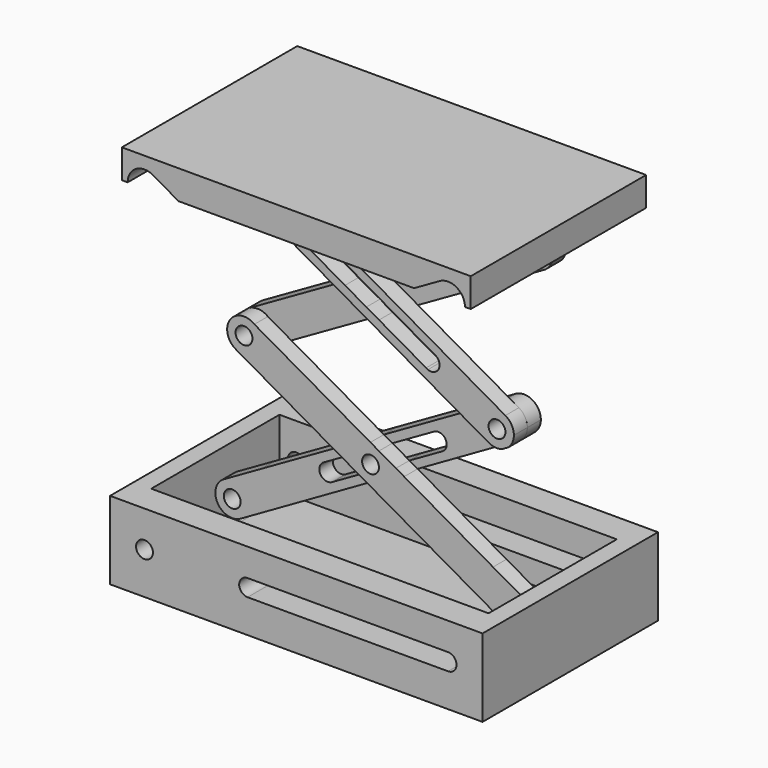
from build123d import *

# Parameters (mm, degrees)
F0_R     = 5
F1_DEPTH = 65
F2_DEPTH = 65
F3_DEPTH = 10
F4_DEPTH = 10
F6_DEPTH = 47.5


# Not quite as in the source:
# - a feature names something its author has since deleted; it is built from what else it names


with BuildPart() as f1:
    # F0 (on Front) → F1 (new body, symmetric)
    with BuildSketch(Plane.XZ):
        with BuildLine():
            Line((-101.2363367384, 45.0652157913), (-79.5725504618, 57.4387013912))
            Line((-79.5725504618, 57.4387013912), (-117.3849242899, 57.4387013912))
            Line((-117.3849242899, 57.4387013912), (-117.3849242899, 11.2442991069))
            Line((-117.3849242899, 11.2442991069), (-6.9597655522, 11.2442991069))
            Line((-6.9597655522, 11.2442991069), (103.4653931856, 11.2442991069))
            Line((103.4653931856, 11.2442991069), (103.4653931856, 57.4387013912))
            Line((103.4653931856, 57.4387013912), (65.6763988632, 57.4387013912))
            Line((65.6763988632, 57.4387013912), (87.9937572054, 44.7127273849))
            ThreePointArc((87.9937572054, 44.7127273849), (91.6870612524, 41.0489903412), (93.0402344479, 36.0258054737))
            ThreePointArc((93.0402344479, 36.0258054737), (87.7852934476, 27.2232822509), (77.54335143, 27.6721070659))
            Line((77.54335143, 27.6721070659), (71.668050416, 31.0258054737))
            Line((71.668050416, 31.0258054737), (-35.829693079, 31.0258054737))
            ThreePointArc((-35.829693079, 31.0258054737), (-40.829693079, 36.0258054737), (-35.829693079, 41.0258054737))
            Line((-35.829693079, 41.0258054737), (54.1491793085, 41.0258054737))
            Line((54.1491793085, 41.0258054737), (25.3956385004, 57.4387013912))
            Line((25.3956385004, 57.4387013912), (-39.4630207883, 57.4387013912))
            Line((-39.4630207883, 57.4387013912), (-91.9890244833, 27.3487245576))
            ThreePointArc((-91.9890244833, 27.3487245576), (-105.4423640429, 30.730003094), (-102.5730303875, 44.3017500052))
            ThreePointArc((-102.5730303875, 44.3017500052), (-101.9193959956, 44.7092417673), (-101.2363367384, 45.0652157913))
        make_face()
        with BuildLine():
            ThreePointArc((93.0402344479, 36.0258054737), (91.6870612524, 41.0489903412), (87.9937572054, 44.7127273849))
            ThreePointArc((87.9937572054, 44.7127273849), (80.4261739109, 45.6780947104), (74.37998041, 41.0258054737))
            Line((74.37998041, 41.0258054737), (83.0402344479, 41.0258054737))
            ThreePointArc((83.0402344479, 41.0258054737), (86.5757683538, 39.5613393797), (88.0402344479, 36.0258054737))
            ThreePointArc((88.0402344479, 36.0258054737), (86.5757683538, 32.4902715678), (83.0402344479, 31.0258054737))
            Line((83.0402344479, 31.0258054737), (74.37998041, 31.0258054737))
            ThreePointArc((74.37998041, 31.0258054737), (75.7657615696, 29.1641697836), (77.54335143, 27.6721070659))
            ThreePointArc((77.54335143, 27.6721070659), (87.7852934476, 27.2232822509), (93.0402344479, 36.0258054737))
        make_face()
        with BuildLine():
            Line((87.9937572054, 44.7127273849), (65.6763988632, 57.4387013912))
            Line((65.6763988632, 57.4387013912), (25.3956385004, 57.4387013912))
            Line((25.3956385004, 57.4387013912), (54.1491793085, 41.0258054737))
            Line((54.1491793085, 41.0258054737), (74.37998041, 41.0258054737))
            ThreePointArc((74.37998041, 41.0258054737), (80.4261739109, 45.6780947104), (87.9937572054, 44.7127273849))
        make_face()
        with BuildLine():
            Line((-39.4630207883, 57.4387013912), (-79.5725504618, 57.4387013912))
            Line((-79.5725504618, 57.4387013912), (-101.2363367384, 45.0652157913))
            ThreePointArc((-101.2363367384, 45.0652157913), (-91.6102661299, 44.4746430228), (-86.9597655521, 36.0258054737))
            ThreePointArc((-86.9597655521, 36.0258054737), (-88.307961963, 31.0111973479), (-91.9890244833, 27.3487245576))
            Line((-91.9890244833, 27.3487245576), (-39.4630207883, 57.4387013912))
        make_face()
        with BuildLine():
            ThreePointArc((-86.9597655521, 36.0258054737), (-91.6102661299, 44.4746430228), (-101.2363367384, 45.0652157913))
            Line((-101.2363367384, 45.0652157913), (-102.5730303875, 44.3017500052))
            ThreePointArc((-102.5730303875, 44.3017500052), (-105.4423640429, 30.730003094), (-91.9890244833, 27.3487245576))
            ThreePointArc((-91.9890244833, 27.3487245576), (-88.307961963, 31.0111973479), (-86.9597655521, 36.0258054737))
        make_face()
        with Locations((-96.9597655521, 36.0258054737)):
            Circle(F0_R, mode=Mode.SUBTRACT)
        with BuildLine():
            Line((74.37998041, 31.0258054737), (71.668050416, 31.0258054737))
            Line((71.668050416, 31.0258054737), (77.54335143, 27.6721070659))
            ThreePointArc((77.54335143, 27.6721070659), (75.7657615696, 29.1641697836), (74.37998041, 31.0258054737))
        make_face()
    extrude(amount=F1_DEPTH, both=True)

    # F5 (on Front) → F6 (cut, symmetric)
    with BuildSketch(Plane.XZ):
        with BuildLine():
            ThreePointArc((-106.9597655522, 22.2442991069), (-105.4296671345, 18.835091297), (-101.9635462063, 17.4387013912))
            Line((-101.9635462063, 17.4387013912), (88.0402344478, 17.4387013912))
            ThreePointArc((88.0402344478, 17.4387013912), (91.5757683538, 18.9031674853), (93.0402344478, 22.4387013912))
            Line((93.0402344478, 22.4387013912), (93.0402344478, 57.4387013912))
            Line((93.0402344478, 57.4387013912), (-106.9597655522, 57.4387013912))
            Line((-106.9597655522, 57.4387013912), (-106.9597655522, 22.2442991069))
        make_face()
    extrude(amount=F6_DEPTH, both=True, mode=Mode.SUBTRACT)


with BuildPart() as f2:
    # F0 (on Front) → F2 (new body, symmetric)
    with BuildSketch(Plane.XZ):
        with BuildLine():
            Line((96.4685455285, 224.4402422879), (96.4685455285, 241.6182321313))
            Line((96.4685455285, 241.6182321313), (-110.3880766328, 241.6182321313))
            Line((-110.3880766328, 241.6182321313), (-110.3880766328, 224.4402422879))
            Line((-110.3880766328, 224.4402422879), (-106.9597655522, 224.4402422879))
            ThreePointArc((-106.9597655522, 224.4402422879), (-101.9805848812, 233.0884428675), (-92.0014908991, 233.1244528142))
            Line((-92.0014908991, 233.1244528142), (-76.7914596396, 224.4402422879))
            Line((-76.7914596396, 224.4402422879), (62.8719285353, 224.4402422879))
            Line((62.8719285353, 224.4402422879), (78.0819597948, 233.1244528142))
            ThreePointArc((78.0819597948, 233.1244528142), (88.0610537769, 233.0884428675), (93.0402344479, 224.4402422879))
            Line((93.0402344479, 224.4402422879), (96.4685455285, 224.4402422879))
        make_face()
    extrude(amount=F2_DEPTH, both=True)


with BuildPart() as f3:
    # F0 (on Front) → F3 (new body)
    with BuildSketch(Plane.XZ):
        with BuildLine():
            ThreePointArc((-92.0014908991, 233.1244528142), (-101.9805848812, 233.0884428675), (-106.9597655522, 224.4402422879))
            Line((-106.9597655522, 224.4402422879), (-101.9597655522, 224.4402422879))
            ThreePointArc((-101.9597655522, 224.4402422879), (-96.9597655522, 229.4402422879), (-91.9597655522, 224.4402422879))
            Line((-91.9597655522, 224.4402422879), (-86.9597655522, 224.4402422879))
            ThreePointArc((-86.9597655522, 224.4402422879), (-88.3115649725, 229.461061617), (-92.0014908991, 233.1244528142))
        make_face()
        with BuildLine():
            Line((-101.9597655522, 224.4402422879), (-106.9597655522, 224.4402422879))
            ThreePointArc((-106.9597655522, 224.4402422879), (-105.6079661318, 219.4194229589), (-101.9180402052, 215.7560317616))
            ThreePointArc((-101.9180402052, 215.7560317616), (-91.9389462231, 215.7920417083), (-86.9597655522, 224.4402422879))
            Line((-86.9597655522, 224.4402422879), (-91.9597655522, 224.4402422879))
            ThreePointArc((-91.9597655522, 224.4402422879), (-96.9597655522, 219.4402422879), (-101.9597655522, 224.4402422879))
        make_face()
        with BuildLine():
            Line((-76.7914596396, 224.4402422879), (-92.0014908991, 233.1244528142))
            ThreePointArc((-92.0014908991, 233.1244528142), (-88.3115649725, 229.461061617), (-86.9597655522, 224.4402422879))
            Line((-86.9597655522, 224.4402422879), (-76.7914596396, 224.4402422879))
        make_face()
        with BuildLine():
            ThreePointArc((-86.9597655522, 224.4402422879), (-91.9389462231, 215.7920417083), (-101.9180402052, 215.7560317616))
            Line((-101.9180402052, 215.7560317616), (-27.1280714647, 173.0544867931))
            Line((-27.1280714647, 173.0544867931), (-22.0713976231, 175.941609078))
            Line((-22.0713976231, 175.941609078), (-56.1556671093, 195.3854510802))
            ThreePointArc((-56.1556671093, 195.3854510802), (-58.0206941441, 202.2068069805), (-51.1989943683, 204.070575831))
            Line((-51.1989943683, 204.070575831), (-12.0018420303, 181.6908504295))
            Line((-12.0018420303, 181.6908504295), (-6.9597655522, 184.5696383083))
            Line((-6.9597655522, 184.5696383083), (-76.7914596396, 224.4402422879))
            Line((-76.7914596396, 224.4402422879), (-86.9597655522, 224.4402422879))
        make_face()
        with BuildLine():
            Line((72.9985091009, 138.9172344071), (13.2085403604, 173.0544867931))
            Line((13.2085403604, 173.0544867931), (8.1664638822, 170.1756989143))
            Line((8.1664638822, 170.1756989143), (31.4786934415, 156.865515268))
            ThreePointArc((31.4786934415, 156.865515268), (33.4813572121, 150.3067776658), (27.0532688851, 147.9177649883))
            ThreePointArc((27.0532688851, 147.9177649883), (26.5220207005, 148.1803905172), (26.0255766165, 148.5040262284))
            Line((26.0255766165, 148.5040262284), (-1.8944506773, 164.4313911853))
            Line((-1.8944506773, 164.4313911853), (-6.9597655521, 161.539335278))
            Line((-6.9597655521, 161.539335278), (47.8746856916, 130.2314496746))
            Line((47.8746856916, 130.2314496746), (63.0806040044, 138.9164601744))
            ThreePointArc((63.0806040044, 138.9164601744), (68.0394538065, 140.2330238503), (72.9985091009, 138.9172344071))
        make_face()
        Polygon((8.1664638822, 170.1756989143), (13.2085403604, 173.0544867931), (-6.9597655522, 184.5696383083), (-12.0018420303, 181.6908504295), align=None)
        Polygon((-22.0713976231, 175.941609078), (-27.1280714647, 173.0544867931), (-6.9597655521, 161.539335278), (-1.8944506773, 164.4313911853), (-9.4274673353, 168.728704518), align=None)
        with BuildLine():
            ThreePointArc((78.0402344479, 130.2330238808), (76.6884350275, 135.2538432099), (72.9985091009, 138.9172344071))
            ThreePointArc((72.9985091009, 138.9172344071), (68.0394538065, 140.2330238503), (63.0806040044, 138.9164601744))
            ThreePointArc((63.0806040044, 138.9164601744), (58.0402344783, 130.2322432394), (63.0819597948, 121.5488133545))
            ThreePointArc((63.0819597948, 121.5488133545), (66.8793294994, 120.3006374757), (70.8621881287, 120.6394542937))
            Line((70.8621881287, 120.6394542937), (74.8884976984, 122.9459606554))
            ThreePointArc((74.8884976984, 122.9459606554), (77.2185412771, 126.2633030157), (78.0402344479, 130.2330238808))
        make_face()
        with Locations((68.0402344479, 130.2330238808)):
            Circle(F0_R, mode=Mode.SUBTRACT)
        with BuildLine():
            ThreePointArc((63.0819597948, 121.5488133545), (58.0402344783, 130.2322432394), (63.0806040044, 138.9164601744))
            Line((63.0806040044, 138.9164601744), (47.8746856916, 130.2314496746))
            Line((47.8746856916, 130.2314496746), (63.0819597948, 121.5488133545))
        make_face()
    extrude(amount=F3_DEPTH)


with BuildPart() as f3b:
    # F0 (on Front) → F3, piece 2 (new body)
    with BuildSketch(Plane.XZ):
        with BuildLine():
            ThreePointArc((-75.8084523259, 138.1172705533), (-81.2415588958, 140.2071994958), (-86.9180402052, 138.9172344071))
            ThreePointArc((-86.9180402052, 138.9172344071), (-91.9597655383, 130.2324966831), (-86.9171245184, 121.5482906045))
            ThreePointArc((-86.9171245184, 121.5482906045), (-81.9597655035, 120.2330238808), (-77.0024065014, 121.5482906528))
            ThreePointArc((-77.0024065014, 121.5482906528), (-73.3118296566, 125.2117486697), (-71.9597655521, 130.2330238808))
            ThreePointArc((-71.9597655521, 130.2330238808), (-72.9732998324, 134.6197577306), (-75.8084523259, 138.1172705533))
        make_face()
        with Locations((-81.9597655521, 130.2330238808)):
            Circle(F0_R, mode=Mode.SUBTRACT)
        with BuildLine():
            Line((-61.8866502182, 130.1786745498), (-75.8084523259, 138.1172705533))
            ThreePointArc((-75.8084523259, 138.1172705533), (-72.9732998324, 134.6197577306), (-71.9597655521, 130.2330238808))
            ThreePointArc((-71.9597655521, 130.2330238808), (-73.3118296566, 125.2117486697), (-77.0024065014, 121.5482906528))
            Line((-77.0024064738, 121.5482906045), (-61.8866502182, 130.1786745498))
        make_face()
        with BuildLine():
            ThreePointArc((-77.0024065014, 121.5482906528), (-81.9597655035, 120.2330238808), (-86.9171245184, 121.5482906045))
            Line((-86.9171245184, 121.5482906045), (-27.1043967074, 87.4064058657))
            Line((-27.1043967074, 87.4064058657), (-7.0073943064, 98.8850073732))
            Line((-7.0073943064, 98.8850073732), (-61.8866502182, 130.1786745498))
            Line((-61.8866502182, 130.1786745498), (-77.0024064738, 121.5482906045))
        make_face()
        Polygon((-7.0073943064, 98.8850073732), (-27.1043967074, 87.4064058657), (-22.0780567084, 84.5373054721), (-9.438903152, 91.7536660756), (-1.9748296463, 96.0153000329), align=None)
        with BuildLine():
            Line((-9.438903152, 91.7536660756), (-22.0780567084, 84.5373054721))
            Line((-22.0780567084, 84.5373054721), (-11.9926690021, 78.7804346986))
            Line((-11.9926690021, 78.7804346986), (-4.4806282957, 83.0694556654))
            ThreePointArc((-4.4806282957, 83.0694556654), (-11.3018707573, 84.9324235403), (-9.438903152, 91.7536660756))
        make_face()
        with BuildLine():
            Line((8.1157318271, 90.2613832364), (-1.9748296463, 96.0153000329))
            Line((-1.9748296463, 96.0153000329), (-9.438903152, 91.7536660756))
            ThreePointArc((-9.438903152, 91.7536660756), (-4.4493560237, 91.7356613373), (-1.9597655521, 87.4115609685))
            ThreePointArc((-1.9597655521, 87.4115609685), (-2.6356652826, 84.9011512691), (-4.4806282957, 83.0694556654))
            Line((-4.4806282957, 83.0694556654), (8.1157318271, 90.2613832364))
        make_face()
        Polygon((65.6763988632, 57.4387013912), (12.9856885063, 87.4843994571), (-7.0916961468, 75.9828955049), (25.3956385004, 57.4387013912), align=None)
        Polygon((-7.0916961468, 75.9828955049), (12.9856885063, 87.4843994571), (8.1157318271, 90.2613832364), (-4.4806282957, 83.0694556654), (-11.9926690021, 78.7804346986), align=None)
        with BuildLine():
            Line((87.9937572054, 44.7127273849), (65.6763988632, 57.4387013912))
            Line((65.6763988632, 57.4387013912), (25.3956385004, 57.4387013912))
            Line((25.3956385004, 57.4387013912), (54.1491793085, 41.0258054737))
            Line((54.1491793085, 41.0258054737), (74.37998041, 41.0258054737))
            ThreePointArc((74.37998041, 41.0258054737), (80.4261739109, 45.6780947104), (87.9937572054, 44.7127273849))
        make_face()
        with BuildLine():
            ThreePointArc((93.0402344479, 36.0258054737), (91.6870612524, 41.0489903412), (87.9937572054, 44.7127273849))
            ThreePointArc((87.9937572054, 44.7127273849), (80.4261739109, 45.6780947104), (74.37998041, 41.0258054737))
            Line((74.37998041, 41.0258054737), (83.0402344479, 41.0258054737))
            ThreePointArc((83.0402344479, 41.0258054737), (86.5757683538, 39.5613393797), (88.0402344479, 36.0258054737))
            ThreePointArc((88.0402344479, 36.0258054737), (86.5757683538, 32.4902715678), (83.0402344479, 31.0258054737))
            Line((83.0402344479, 31.0258054737), (74.37998041, 31.0258054737))
            ThreePointArc((74.37998041, 31.0258054737), (75.7657615696, 29.1641697836), (77.54335143, 27.6721070659))
            ThreePointArc((77.54335143, 27.6721070659), (87.7852934476, 27.2232822509), (93.0402344479, 36.0258054737))
        make_face()
        with BuildLine():
            Line((74.37998041, 41.0258054737), (54.1491793085, 41.0258054737))
            Line((54.1491793085, 41.0258054737), (71.668050416, 31.0258054737))
            Line((71.668050416, 31.0258054737), (74.37998041, 31.0258054737))
            ThreePointArc((74.37998041, 31.0258054737), (73.0402344479, 36.0258054737), (74.37998041, 41.0258054737))
        make_face()
        with BuildLine():
            Line((83.0402344479, 41.0258054737), (74.37998041, 41.0258054737))
            ThreePointArc((74.37998041, 41.0258054737), (73.0402344479, 36.0258054737), (74.37998041, 31.0258054737))
            Line((74.37998041, 31.0258054737), (83.0402344479, 31.0258054737))
            ThreePointArc((83.0402344479, 31.0258054737), (78.0402344479, 36.0258054737), (83.0402344479, 41.0258054737))
        make_face()
        with BuildLine():
            Line((74.37998041, 31.0258054737), (71.668050416, 31.0258054737))
            Line((71.668050416, 31.0258054737), (77.54335143, 27.6721070659))
            ThreePointArc((77.54335143, 27.6721070659), (75.7657615696, 29.1641697836), (74.37998041, 31.0258054737))
        make_face()
    extrude(amount=F3_DEPTH)


with BuildPart() as f4:
    # F0 (on Front) → F4 (new body)
    with BuildSketch(Plane.XZ):
        with BuildLine():
            Line((13.2085403604, 173.0544867931), (87.9985091009, 215.7560317616))
            ThreePointArc((87.9985091009, 215.7560317616), (78.0194151188, 215.7920417083), (73.0402344479, 224.4402422879))
            Line((73.0402344479, 224.4402422879), (62.8719285353, 224.4402422879))
            Line((62.8719285353, 224.4402422879), (-6.9597655522, 184.5696383083))
            Line((-6.9597655522, 184.5696383083), (13.2085403604, 173.0544867931))
        make_face()
        with BuildLine():
            ThreePointArc((87.9985091009, 215.7560317616), (91.6884350275, 219.4194229589), (93.0402344479, 224.4402422879))
            Line((93.0402344479, 224.4402422879), (88.0402344479, 224.4402422879))
            ThreePointArc((88.0402344479, 224.4402422879), (83.0402344479, 219.4402422879), (78.0402344479, 224.4402422879))
            Line((78.0402344479, 224.4402422879), (73.0402344479, 224.4402422879))
            ThreePointArc((73.0402344479, 224.4402422879), (78.0194151188, 215.7920417083), (87.9985091009, 215.7560317616))
        make_face()
        with BuildLine():
            Line((88.0402344479, 224.4402422879), (93.0402344479, 224.4402422879))
            ThreePointArc((93.0402344479, 224.4402422879), (88.0610537769, 233.0884428675), (78.0819597948, 233.1244528142))
            ThreePointArc((78.0819597948, 233.1244528142), (74.3920338682, 229.461061617), (73.0402344479, 224.4402422879))
            Line((73.0402344479, 224.4402422879), (78.0402344479, 224.4402422879))
            ThreePointArc((78.0402344479, 224.4402422879), (83.0402344479, 229.4402422879), (88.0402344479, 224.4402422879))
        make_face()
        with BuildLine():
            ThreePointArc((73.0402344479, 224.4402422879), (74.3920338682, 229.461061617), (78.0819597948, 233.1244528142))
            Line((78.0819597948, 233.1244528142), (62.8719285353, 224.4402422879))
            Line((62.8719285353, 224.4402422879), (73.0402344479, 224.4402422879))
        make_face()
        Polygon((8.1664638822, 170.1756989143), (13.2085403604, 173.0544867931), (-6.9597655522, 184.5696383083), (-12.0018420303, 181.6908504295), align=None)
        with BuildLine():
            Line((-6.9597655521, 161.539335278), (-27.1280714647, 173.0544867931))
            Line((-27.1280714647, 173.0544867931), (-86.9180402052, 138.9172344071))
            ThreePointArc((-86.9180402052, 138.9172344071), (-81.2415588958, 140.2071994958), (-75.8084523259, 138.1172705533))
            Line((-75.8084523259, 138.1172705533), (-61.8866502182, 130.1786745498))
            Line((-61.8866502182, 130.1786745498), (-6.9597655521, 161.539335278))
        make_face()
        with BuildLine():
            Line((-61.8866502182, 130.1786745498), (-75.8084523259, 138.1172705533))
            ThreePointArc((-75.8084523259, 138.1172705533), (-72.9732998324, 134.6197577306), (-71.9597655521, 130.2330238808))
            ThreePointArc((-71.9597655521, 130.2330238808), (-73.3118296566, 125.2117486697), (-77.0024065014, 121.5482906528))
            Line((-77.0024064738, 121.5482906045), (-61.8866502182, 130.1786745498))
        make_face()
        with BuildLine():
            ThreePointArc((-75.8084523259, 138.1172705533), (-81.2415588958, 140.2071994958), (-86.9180402052, 138.9172344071))
            ThreePointArc((-86.9180402052, 138.9172344071), (-91.9597655383, 130.2324966831), (-86.9171245184, 121.5482906045))
            ThreePointArc((-86.9171245184, 121.5482906045), (-81.9597655035, 120.2330238808), (-77.0024065014, 121.5482906528))
            ThreePointArc((-77.0024065014, 121.5482906528), (-73.3118296566, 125.2117486697), (-71.9597655521, 130.2330238808))
            ThreePointArc((-71.9597655521, 130.2330238808), (-72.9732998324, 134.6197577306), (-75.8084523259, 138.1172705533))
        make_face()
        with Locations((-81.9597655521, 130.2330238808)):
            Circle(F0_R, mode=Mode.SUBTRACT)
        Polygon((-22.0713976231, 175.941609078), (-27.1280714647, 173.0544867931), (-6.9597655521, 161.539335278), (-1.8944506773, 164.4313911853), (-9.4274673353, 168.728704518), align=None)
        Polygon((-1.8944506773, 164.4313911853), (8.1664638822, 170.1756989143), (-12.0018420303, 181.6908504295), (-22.0713976231, 175.941609078), (-9.4274673353, 168.728704518), align=None)
        with BuildLine():
            ThreePointArc((-1.9796104961, 173.0544867931), (-4.4585251728, 168.7480101652), (-9.4274673353, 168.728704518))
            ThreePointArc((-9.4274673353, 168.728704518), (-9.4610059315, 177.3609634211), (-1.9796104961, 173.0544867931))
        make_face(mode=Mode.SUBTRACT)
    extrude(amount=-F4_DEPTH)


with BuildPart() as f4b:
    # F0 (on Front) → F4, piece 2 (new body)
    with BuildSketch(Plane.XZ):
        with BuildLine():
            Line((63.0819597948, 121.5488133545), (47.8746856916, 130.2314496746))
            Line((47.8746856916, 130.2314496746), (-7.0073943064, 98.8850073732))
            Line((-7.0073943064, 98.8850073732), (-1.9748296463, 96.0153000329))
            Line((-1.9748296463, 96.0153000329), (22.7454364945, 110.1294061627))
            ThreePointArc((22.7454364945, 110.1294061627), (29.5666790842, 108.266438226), (27.7037111475, 101.4451956364))
            Line((27.7037111475, 101.4451956364), (8.1157318271, 90.2613832364))
            Line((8.1157318271, 90.2613832364), (12.9856885063, 87.4843994571))
            Line((12.9856885063, 87.4843994571), (70.8621881287, 120.6394542937))
            ThreePointArc((70.8621881287, 120.6394542937), (66.8793294994, 120.3006374757), (63.0819597948, 121.5488133545))
        make_face()
        with BuildLine():
            ThreePointArc((78.0402344479, 130.2330238808), (76.6884350275, 135.2538432099), (72.9985091009, 138.9172344071))
            ThreePointArc((72.9985091009, 138.9172344071), (68.0394538065, 140.2330238503), (63.0806040044, 138.9164601744))
            ThreePointArc((63.0806040044, 138.9164601744), (58.0402344783, 130.2322432394), (63.0819597948, 121.5488133545))
            ThreePointArc((63.0819597948, 121.5488133545), (66.8793294994, 120.3006374757), (70.8621881287, 120.6394542937))
            Line((70.8621881287, 120.6394542937), (74.8884976984, 122.9459606554))
            ThreePointArc((74.8884976984, 122.9459606554), (77.2185412771, 126.2633030157), (78.0402344479, 130.2330238808))
        make_face()
        with Locations((68.0402344479, 130.2330238808)):
            Circle(F0_R, mode=Mode.SUBTRACT)
        with BuildLine():
            ThreePointArc((63.0819597948, 121.5488133545), (58.0402344783, 130.2322432394), (63.0806040044, 138.9164601744))
            Line((63.0806040044, 138.9164601744), (47.8746856916, 130.2314496746))
            Line((47.8746856916, 130.2314496746), (63.0819597948, 121.5488133545))
        make_face()
        Polygon((-7.0073943064, 98.8850073732), (-27.1043967074, 87.4064058657), (-22.0780567084, 84.5373054721), (-9.438903152, 91.7536660756), (-1.9748296463, 96.0153000329), align=None)
        Polygon((-7.0916961468, 75.9828955049), (12.9856885063, 87.4843994571), (8.1157318271, 90.2613832364), (-4.4806282957, 83.0694556654), (-11.9926690021, 78.7804346986), align=None)
        with BuildLine():
            Line((-22.0780567084, 84.5373054721), (-27.1043967074, 87.4064058657))
            Line((-27.1043967074, 87.4064058657), (-79.5725504618, 57.4387013912))
            Line((-79.5725504618, 57.4387013912), (-39.4630207883, 57.4387013912))
            Line((-39.4630207883, 57.4387013912), (-7.0916961468, 75.9828955049))
            Line((-7.0916961468, 75.9828955049), (-11.9926690021, 78.7804346986))
            Line((-11.9926690021, 78.7804346986), (-37.8288387088, 64.0292002601))
            ThreePointArc((-37.8288387088, 64.0292002601), (-44.6500812985, 65.8921681967), (-42.7871133618, 72.7134107864))
            Line((-42.7871133618, 72.7134107864), (-22.0780567084, 84.5373054721))
        make_face()
        with BuildLine():
            Line((-39.4630207883, 57.4387013912), (-79.5725504618, 57.4387013912))
            Line((-79.5725504618, 57.4387013912), (-101.2363367384, 45.0652157913))
            ThreePointArc((-101.2363367384, 45.0652157913), (-91.6102661299, 44.4746430228), (-86.9597655521, 36.0258054737))
            ThreePointArc((-86.9597655521, 36.0258054737), (-88.307961963, 31.0111973479), (-91.9890244833, 27.3487245576))
            Line((-91.9890244833, 27.3487245576), (-39.4630207883, 57.4387013912))
        make_face()
        with BuildLine():
            ThreePointArc((-86.9597655521, 36.0258054737), (-91.6102661299, 44.4746430228), (-101.2363367384, 45.0652157913))
            Line((-101.2363367384, 45.0652157913), (-102.5730303875, 44.3017500052))
            ThreePointArc((-102.5730303875, 44.3017500052), (-105.4423640429, 30.730003094), (-91.9890244833, 27.3487245576))
            ThreePointArc((-91.9890244833, 27.3487245576), (-88.307961963, 31.0111973479), (-86.9597655521, 36.0258054737))
        make_face()
        with Locations((-96.9597655521, 36.0258054737)):
            Circle(F0_R, mode=Mode.SUBTRACT)
    extrude(amount=-F4_DEPTH)


solid = Compound([f1.part, f2.part, f3.part, f3b.part, f4.part, f4b.part])
